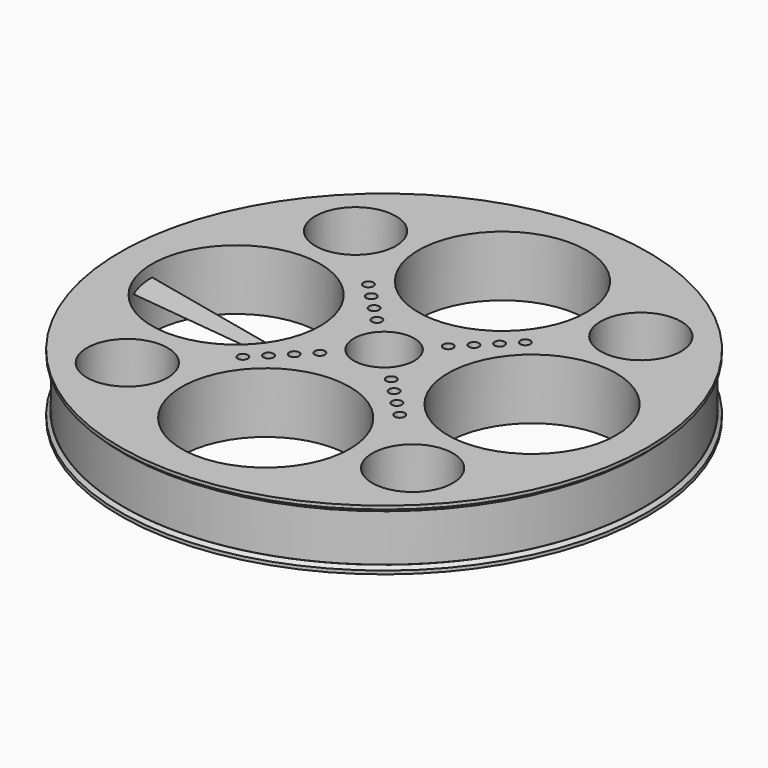
from build123d import *

# Parameters (mm, degrees)
F0_R     = 38.7121
F0_R_2   = 6
F0_R_3   = 0.75
F0_R_4   = 12.5
F0_R_5   = 4.5
F1_DEPTH = 7
F2_R     = 39.25
F2_R_2   = 38.7121
F2_R_3   = 6
F2_R_4   = 0.75
F2_R_5   = 12.5
F2_R_6   = 4.5
F3_DEPTH = 1
F4_R     = 39.25
F4_R_2   = 38.7121
F4_R_3   = 6
F4_R_4   = 0.75
F4_R_5   = 12.5
F4_R_6   = 4.5
F5_DEPTH = 1
F6_SIZE  = 0.5


with BuildPart() as f1:
    # F0 (on Top) → F1 (new body)
    with BuildSketch(Plane.XY):
        Circle(F0_R)
        with Locations((-21.2132034356, -21.2132034356)):
            Circle(F0_R_2, mode=Mode.SUBTRACT)
        with Locations((-11.6672618896, -11.6672618896)):
            Circle(F0_R_3, mode=Mode.SUBTRACT)
        with Locations((-9.545941546, -9.545941546)):
            Circle(F0_R_3, mode=Mode.SUBTRACT)
        with Locations((-7.4246212025, -7.4246212025)):
            Circle(F0_R_3, mode=Mode.SUBTRACT)
        with Locations((-5.3033008589, -5.3033008589)):
            Circle(F0_R_3, mode=Mode.SUBTRACT)
        with Locations((0, -22)):
            Circle(F0_R_4, mode=Mode.SUBTRACT)
        with Locations((21.2132034356, -21.2132034356)):
            Circle(F0_R_2, mode=Mode.SUBTRACT)
        with Locations((11.6672618896, -11.6672618896)):
            Circle(F0_R_3, mode=Mode.SUBTRACT)
        with Locations((9.545941546, -9.545941546)):
            Circle(F0_R_3, mode=Mode.SUBTRACT)
        with Locations((7.4246212025, -7.4246212025)):
            Circle(F0_R_3, mode=Mode.SUBTRACT)
        with Locations((5.3033008589, -5.3033008589)):
            Circle(F0_R_3, mode=Mode.SUBTRACT)
        with Locations((-22, 0)):
            Circle(F0_R_4, mode=Mode.SUBTRACT)
        with Locations((-5.3033008589, 5.3033008589)):
            Circle(F0_R_3, mode=Mode.SUBTRACT)
        with Locations((-7.4246212025, 7.4246212025)):
            Circle(F0_R_3, mode=Mode.SUBTRACT)
        with Locations((-9.545941546, 9.545941546)):
            Circle(F0_R_3, mode=Mode.SUBTRACT)
        with Locations((-11.6672618896, 11.6672618896)):
            Circle(F0_R_3, mode=Mode.SUBTRACT)
        with Locations((-21.2132034356, 21.2132034356)):
            Circle(F0_R_2, mode=Mode.SUBTRACT)
        Circle(F0_R_5, mode=Mode.SUBTRACT)
        with Locations((5.3033008589, 5.3033008589)):
            Circle(F0_R_3, mode=Mode.SUBTRACT)
        with Locations((7.4246212025, 7.4246212025)):
            Circle(F0_R_3, mode=Mode.SUBTRACT)
        with Locations((9.545941546, 9.545941546)):
            Circle(F0_R_3, mode=Mode.SUBTRACT)
        with Locations((11.6672618896, 11.6672618896)):
            Circle(F0_R_3, mode=Mode.SUBTRACT)
        with Locations((22, 0)):
            Circle(F0_R_4, mode=Mode.SUBTRACT)
        with Locations((0, 22)):
            Circle(F0_R_4, mode=Mode.SUBTRACT)
        with Locations((21.2132034356, 21.2132034356)):
            Circle(F0_R_2, mode=Mode.SUBTRACT)
    extrude(amount=F1_DEPTH)

    # F2 (on face) → F3 (join)
    with BuildSketch(Plane.XY.offset(7)):
        Circle(F2_R)
        Circle(F2_R_2, mode=Mode.SUBTRACT)
        Circle(F2_R_2)
        with Locations((-21.2132034356, -21.2132034356)):
            Circle(F2_R_3, mode=Mode.SUBTRACT)
        with Locations((-11.6672618896, -11.6672618896)):
            Circle(F2_R_4, mode=Mode.SUBTRACT)
        with Locations((-9.545941546, -9.545941546)):
            Circle(F2_R_4, mode=Mode.SUBTRACT)
        with Locations((-7.4246212025, -7.4246212025)):
            Circle(F2_R_4, mode=Mode.SUBTRACT)
        with Locations((-5.3033008589, -5.3033008589)):
            Circle(F2_R_4, mode=Mode.SUBTRACT)
        with Locations((0, -22)):
            Circle(F2_R_5, mode=Mode.SUBTRACT)
        with Locations((21.2132034356, -21.2132034356)):
            Circle(F2_R_3, mode=Mode.SUBTRACT)
        with Locations((11.6672618896, -11.6672618896)):
            Circle(F2_R_4, mode=Mode.SUBTRACT)
        with Locations((9.545941546, -9.545941546)):
            Circle(F2_R_4, mode=Mode.SUBTRACT)
        with Locations((7.4246212025, -7.4246212025)):
            Circle(F2_R_4, mode=Mode.SUBTRACT)
        with Locations((5.3033008589, -5.3033008589)):
            Circle(F2_R_4, mode=Mode.SUBTRACT)
        with Locations((-22, 0)):
            Circle(F2_R_5, mode=Mode.SUBTRACT)
        with Locations((-5.3033008589, 5.3033008589)):
            Circle(F2_R_4, mode=Mode.SUBTRACT)
        with Locations((-7.4246212025, 7.4246212025)):
            Circle(F2_R_4, mode=Mode.SUBTRACT)
        with Locations((-9.545941546, 9.545941546)):
            Circle(F2_R_4, mode=Mode.SUBTRACT)
        with Locations((-11.6672618896, 11.6672618896)):
            Circle(F2_R_4, mode=Mode.SUBTRACT)
        with Locations((-21.2132034356, 21.2132034356)):
            Circle(F2_R_3, mode=Mode.SUBTRACT)
        Circle(F2_R_6, mode=Mode.SUBTRACT)
        with Locations((5.3033008589, 5.3033008589)):
            Circle(F2_R_4, mode=Mode.SUBTRACT)
        with Locations((7.4246212025, 7.4246212025)):
            Circle(F2_R_4, mode=Mode.SUBTRACT)
        with Locations((9.545941546, 9.545941546)):
            Circle(F2_R_4, mode=Mode.SUBTRACT)
        with Locations((11.6672618896, 11.6672618896)):
            Circle(F2_R_4, mode=Mode.SUBTRACT)
        with Locations((22, 0)):
            Circle(F2_R_5, mode=Mode.SUBTRACT)
        with Locations((0, 22)):
            Circle(F2_R_5, mode=Mode.SUBTRACT)
        with Locations((21.2132034356, 21.2132034356)):
            Circle(F2_R_3, mode=Mode.SUBTRACT)
    extrude(amount=F3_DEPTH)

    # F4 (on face) → F5 (join)
    with BuildSketch(Plane(origin=(0, 0, 0), x_dir=(1, 0, 0), z_dir=(0, 0, -1))):
        Circle(F4_R)
        Circle(F4_R_2, mode=Mode.SUBTRACT)
        Circle(F4_R_2)
        with Locations((-21.2132034356, -21.2132034356)):
            Circle(F4_R_3, mode=Mode.SUBTRACT)
        with Locations((-11.6672618896, -11.6672618896)):
            Circle(F4_R_4, mode=Mode.SUBTRACT)
        with Locations((-9.545941546, -9.545941546)):
            Circle(F4_R_4, mode=Mode.SUBTRACT)
        with Locations((-7.4246212025, -7.4246212025)):
            Circle(F4_R_4, mode=Mode.SUBTRACT)
        with Locations((-5.3033008589, -5.3033008589)):
            Circle(F4_R_4, mode=Mode.SUBTRACT)
        with Locations((0, -22)):
            Circle(F4_R_5, mode=Mode.SUBTRACT)
        with Locations((21.2132034356, -21.2132034356)):
            Circle(F4_R_3, mode=Mode.SUBTRACT)
        with Locations((11.6672618896, -11.6672618896)):
            Circle(F4_R_4, mode=Mode.SUBTRACT)
        with Locations((9.545941546, -9.545941546)):
            Circle(F4_R_4, mode=Mode.SUBTRACT)
        with Locations((7.4246212025, -7.4246212025)):
            Circle(F4_R_4, mode=Mode.SUBTRACT)
        with Locations((5.3033008589, -5.3033008589)):
            Circle(F4_R_4, mode=Mode.SUBTRACT)
        with Locations((-22, 0)):
            Circle(F4_R_5, mode=Mode.SUBTRACT)
        with Locations((-5.3033008589, 5.3033008589)):
            Circle(F4_R_4, mode=Mode.SUBTRACT)
        with Locations((-7.4246212025, 7.4246212025)):
            Circle(F4_R_4, mode=Mode.SUBTRACT)
        with Locations((-9.545941546, 9.545941546)):
            Circle(F4_R_4, mode=Mode.SUBTRACT)
        with Locations((-11.6672618896, 11.6672618896)):
            Circle(F4_R_4, mode=Mode.SUBTRACT)
        with Locations((-21.2132034356, 21.2132034356)):
            Circle(F4_R_3, mode=Mode.SUBTRACT)
        Circle(F4_R_6, mode=Mode.SUBTRACT)
        with Locations((5.3033008589, 5.3033008589)):
            Circle(F4_R_4, mode=Mode.SUBTRACT)
        with Locations((7.4246212025, 7.4246212025)):
            Circle(F4_R_4, mode=Mode.SUBTRACT)
        with Locations((9.545941546, 9.545941546)):
            Circle(F4_R_4, mode=Mode.SUBTRACT)
        with Locations((11.6672618896, 11.6672618896)):
            Circle(F4_R_4, mode=Mode.SUBTRACT)
        with Locations((22, 0)):
            Circle(F4_R_5, mode=Mode.SUBTRACT)
        with Locations((0, 22)):
            Circle(F4_R_5, mode=Mode.SUBTRACT)
        with Locations((21.2132034356, 21.2132034356)):
            Circle(F4_R_3, mode=Mode.SUBTRACT)
    extrude(amount=F5_DEPTH)

    # F6
    f6_edges = [f1.edges().sort_by_distance(p)[0] for p in [
        (-39.25, 0, 0),
        (-39.25, 0, 7),
    ]]
    chamfer(f6_edges, length=F6_SIZE)


solid = f1.part
